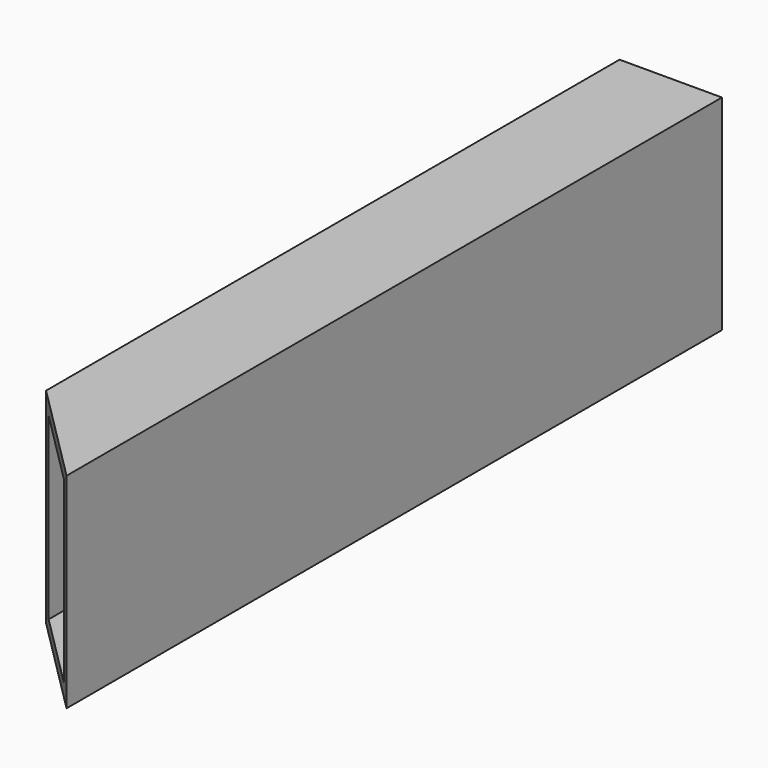
from build123d import *

# Parameters (mm, degrees)
F0_W        = 25.4
F0_H        = 50.8
F0_W_2      = 19.05
F0_H_2      = 44.45
F1_DEPTH    = 203.2
F2_T1_DEPTH = 181.4414957887


# Not quite as in the source:
# - a fillet or chamfer that OpenCascade refuses, or shapes differently, is made with other operations: its cross-section is extruded or revolved along the edge and cut away or added


with BuildPart() as f1:
    # F0 (on Front) → F1 (new body)
    with BuildSketch(Plane.XZ):
        with Locations((0, 11.1125)):
            Rectangle(F0_W, F0_H)
        with Locations((0, 11.1125)):
            Rectangle(F0_W_2, F0_H_2, mode=Mode.SUBTRACT)
    extrude(amount=F1_DEPTH)

    # F2: chamfer of 25.4 on 1 edges, made by hand

    # F2_s2 → F2_t1 (cut)
    with BuildSketch(Plane.XY.offset(-79.6082478943)):
        Polygon((-12.7, -177.8), (12.7, -203.2), (-12.7, -203.2), align=None)
    extrude(amount=F2_T1_DEPTH, mode=Mode.SUBTRACT)


solid = f1.part
